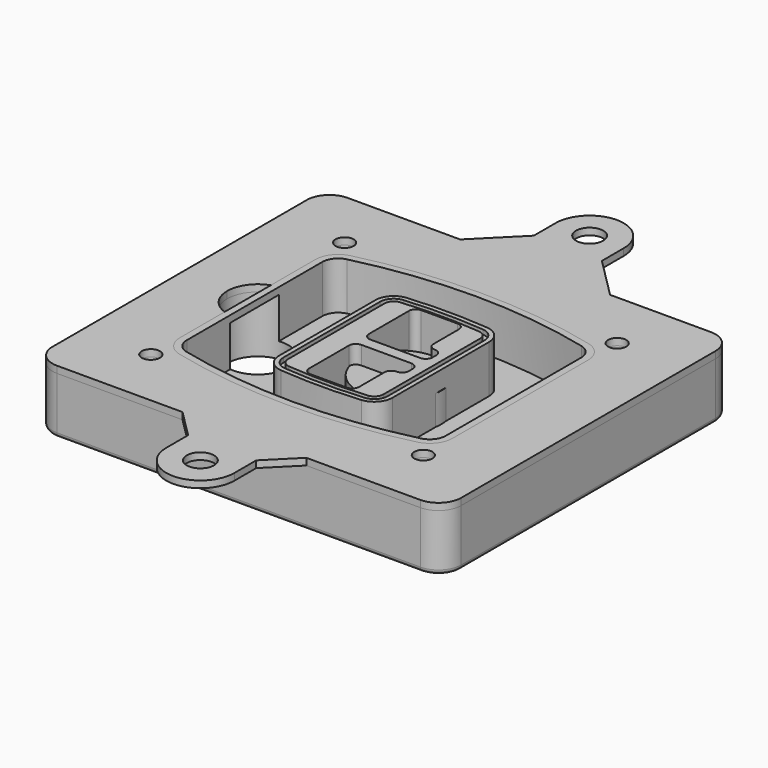
from build123d import *

# Parameters (mm, degrees)
F0_R      = 4
F1_DEPTH  = 25
F2_DEPTH  = 3
F3_DEPTH  = 18
F5_DEPTH  = 21
F6_DEPTH  = 2
F8_DEPTH  = 20
F9_DEPTH  = 16
F10_DEPTH = 25
F7_R      = 6
F7_R_2    = 4
F11_DEPTH = 6
F13_DEPTH = 9
F15_R     = 2
F16_R     = 6
F16_R_2   = 4
F17_DEPTH = 3


# Not quite as in the source:
# - a feature of the source that left no trace in its solid (it failed there, or was rolled back) is left out
# - a feature names something its author has since deleted; it is built from what else it names


with BuildPart() as f1:
    # F0 (on Top) → F1 (new body)
    with BuildSketch(Plane.XY):
        with BuildLine():
            ThreePointArc((-90, -70), (-87.0710678119, -77.0710678119), (-80, -80))
            Line((-80, -80), (80, -80))
            ThreePointArc((80, -80), (87.0710678119, -77.0710678119), (90, -70))
            Line((90, -70), (90, 70))
            ThreePointArc((90, 70), (87.0710678119, 77.0710678119), (80, 80))
            Line((80, 80), (-80, 80))
            ThreePointArc((-80, 80), (-87.0710678119, 77.0710678119), (-90, 70))
            Line((-90, 70), (-90, -70))
        make_face()
        with Locations((-60, -53.3333333333)):
            Circle(F0_R, mode=Mode.SUBTRACT)
        with Locations((60, -53.3333333333)):
            Circle(F0_R, mode=Mode.SUBTRACT)
        with Locations((-60, 53.3333333333)):
            Circle(F0_R, mode=Mode.SUBTRACT)
        with BuildLine():
            ThreePointArc((-64, 37.2990447398), (-61.0143011354, 45.9411029726), (-53.3306899286, 50.8970778549))
            ThreePointArc((-53.3306899286, 50.8970778549), (0, 57.3333333333), (53.3306899286, 50.8970778549))
            ThreePointArc((53.3306899286, 50.8970778549), (61.0143011354, 45.9411029726), (64, 37.2990447398))
            Line((64, 37.2990447398), (64, -37.2990447398))
            ThreePointArc((64, -37.2990447398), (61.0143011354, -45.9411029726), (53.3306899286, -50.8970778549))
            ThreePointArc((53.3306899286, -50.8970778549), (0, -57.3333333333), (-53.3306899286, -50.8970778549))
            ThreePointArc((-53.3306899286, -50.8970778549), (-61.0143011354, -45.9411029726), (-64, -37.2990447398))
            Line((-64, -37.2990447398), (-64, 37.2990447398))
        make_face(mode=Mode.SUBTRACT)
        with Locations((60, 53.3333333333)):
            Circle(F0_R, mode=Mode.SUBTRACT)
        with BuildLine():
            ThreePointArc((53.3306899286, 50.8970778549), (0, 57.3333333333), (-53.3306899286, 50.8970778549))
            ThreePointArc((-53.3306899286, 50.8970778549), (-61.0143011354, 45.9411029726), (-64, 37.2990447398))
            Line((-64, 37.2990447398), (-64, -37.2990447398))
            ThreePointArc((-64, -37.2990447398), (-61.0143011354, -45.9411029726), (-53.3306899286, -50.8970778549))
            ThreePointArc((-53.3306899286, -50.8970778549), (0, -57.3333333333), (53.3306899286, -50.8970778549))
            ThreePointArc((53.3306899286, -50.8970778549), (61.0143011354, -45.9411029726), (64, -37.2990447398))
            Line((64, -37.2990447398), (64, 37.2990447398))
            ThreePointArc((64, 37.2990447398), (61.0143011354, 45.9411029726), (53.3306899286, 50.8970778549))
        make_face()
        with BuildLine():
            Line((-60, -37.2990447398), (-60, 37.2990447398))
            ThreePointArc((-60, 37.2990447398), (-57.8673579538, 43.4719434775), (-52.3790642347, 47.0119255363))
            ThreePointArc((-52.3790642347, 47.0119255363), (0, 53.3333333333), (52.3790642347, 47.0119255363))
            ThreePointArc((52.3790642347, 47.0119255363), (57.8673579538, 43.4719434775), (60, 37.2990447398))
            Line((60, 37.2990447398), (60, -37.2990447398))
            ThreePointArc((60, -37.2990447398), (57.8673579538, -43.4719434775), (52.3790642347, -47.0119255363))
            ThreePointArc((52.3790642347, -47.0119255363), (0, -53.3333333333), (-52.3790642347, -47.0119255363))
            ThreePointArc((-52.3790642347, -47.0119255363), (-57.8673579538, -43.4719434775), (-60, -37.2990447398))
        make_face(mode=Mode.SUBTRACT)
        with BuildLine():
            ThreePointArc((-52.3790642347, 47.0119255363), (-57.8673579538, 43.4719434775), (-60, 37.2990447398))
            Line((-60, 37.2990447398), (-60, -37.2990447398))
            ThreePointArc((-60, -37.2990447398), (-57.8673579538, -43.4719434775), (-52.3790642347, -47.0119255363))
            ThreePointArc((-52.3790642347, -47.0119255363), (0, -53.3333333333), (52.3790642347, -47.0119255363))
            ThreePointArc((52.3790642347, -47.0119255363), (57.8673579538, -43.4719434775), (60, -37.2990447398))
            Line((60, -37.2990447398), (60, 37.2990447398))
            ThreePointArc((60, 37.2990447398), (57.8673579538, 43.4719434775), (52.3790642347, 47.0119255363))
            ThreePointArc((52.3790642347, 47.0119255363), (0, 53.3333333333), (-52.3790642347, 47.0119255363))
        make_face()
        with BuildLine():
            ThreePointArc((51.6653449643, 44.0980612973), (55.5071505677, 41.6200738562), (57, 37.2990447398))
            Line((57, 37.2990447398), (57, -37.2990447398))
            ThreePointArc((57, -37.2990447398), (55.5071505677, -41.6200738562), (51.6653449643, -44.0980612973))
            ThreePointArc((51.6653449643, -44.0980612973), (0, -50.3333333333), (-51.6653449643, -44.0980612973))
            ThreePointArc((-51.6653449643, -44.0980612973), (-55.5071505677, -41.6200738562), (-57, -37.2990447398))
            Line((-57, -37.2990447398), (-57, 37.2990447398))
            ThreePointArc((-57, 37.2990447398), (-55.5071505677, 41.6200738562), (-51.6653449643, 44.0980612973))
            ThreePointArc((-51.6653449643, 44.0980612973), (0, 50.3333333333), (51.6653449643, 44.0980612973))
        make_face(mode=Mode.SUBTRACT)
        with BuildLine():
            Line((57, -37.2990447398), (57, 37.2990447398))
            ThreePointArc((57, 37.2990447398), (55.5071505677, 41.6200738562), (51.6653449643, 44.0980612973))
            ThreePointArc((51.6653449643, 44.0980612973), (0, 50.3333333333), (-51.6653449643, 44.0980612973))
            ThreePointArc((-51.6653449643, 44.0980612973), (-55.5071505677, 41.6200738562), (-57, 37.2990447398))
            Line((-57, 37.2990447398), (-57, -37.2990447398))
            ThreePointArc((-57, -37.2990447398), (-55.5071505677, -41.6200738562), (-51.6653449643, -44.0980612973))
            ThreePointArc((-51.6653449643, -44.0980612973), (0, -50.3333333333), (51.6653449643, -44.0980612973))
            ThreePointArc((51.6653449643, -44.0980612973), (55.5071505677, -41.6200738562), (57, -37.2990447398))
        make_face()
    extrude(amount=-F1_DEPTH)

    # F0 (on Top) → F2 (join)
    with BuildSketch(Plane.XY):
        with BuildLine():
            ThreePointArc((-52.3790642347, 47.0119255363), (-57.8673579538, 43.4719434775), (-60, 37.2990447398))
            Line((-60, 37.2990447398), (-60, -37.2990447398))
            ThreePointArc((-60, -37.2990447398), (-57.8673579538, -43.4719434775), (-52.3790642347, -47.0119255363))
            ThreePointArc((-52.3790642347, -47.0119255363), (0, -53.3333333333), (52.3790642347, -47.0119255363))
            ThreePointArc((52.3790642347, -47.0119255363), (57.8673579538, -43.4719434775), (60, -37.2990447398))
            Line((60, -37.2990447398), (60, 37.2990447398))
            ThreePointArc((60, 37.2990447398), (57.8673579538, 43.4719434775), (52.3790642347, 47.0119255363))
            ThreePointArc((52.3790642347, 47.0119255363), (0, 53.3333333333), (-52.3790642347, 47.0119255363))
        make_face()
        with BuildLine():
            ThreePointArc((51.6653449643, 44.0980612973), (55.5071505677, 41.6200738562), (57, 37.2990447398))
            Line((57, 37.2990447398), (57, -37.2990447398))
            ThreePointArc((57, -37.2990447398), (55.5071505677, -41.6200738562), (51.6653449643, -44.0980612973))
            ThreePointArc((51.6653449643, -44.0980612973), (0, -50.3333333333), (-51.6653449643, -44.0980612973))
            ThreePointArc((-51.6653449643, -44.0980612973), (-55.5071505677, -41.6200738562), (-57, -37.2990447398))
            Line((-57, -37.2990447398), (-57, 37.2990447398))
            ThreePointArc((-57, 37.2990447398), (-55.5071505677, 41.6200738562), (-51.6653449643, 44.0980612973))
            ThreePointArc((-51.6653449643, 44.0980612973), (0, 50.3333333333), (51.6653449643, 44.0980612973))
        make_face(mode=Mode.SUBTRACT)
    extrude(amount=F2_DEPTH)

    # F0 (on Top) → F3 (cut)
    with BuildSketch(Plane.XY):
        with BuildLine():
            Line((57, -37.2990447398), (57, 37.2990447398))
            ThreePointArc((57, 37.2990447398), (55.5071505677, 41.6200738562), (51.6653449643, 44.0980612973))
            ThreePointArc((51.6653449643, 44.0980612973), (0, 50.3333333333), (-51.6653449643, 44.0980612973))
            ThreePointArc((-51.6653449643, 44.0980612973), (-55.5071505677, 41.6200738562), (-57, 37.2990447398))
            Line((-57, 37.2990447398), (-57, -37.2990447398))
            ThreePointArc((-57, -37.2990447398), (-55.5071505677, -41.6200738562), (-51.6653449643, -44.0980612973))
            ThreePointArc((-51.6653449643, -44.0980612973), (0, -50.3333333333), (51.6653449643, -44.0980612973))
            ThreePointArc((51.6653449643, -44.0980612973), (55.5071505677, -41.6200738562), (57, -37.2990447398))
        make_face()
    extrude(amount=-F3_DEPTH, mode=Mode.SUBTRACT)

    # F4 (on face) → F5 (join, through all)
    with BuildSketch(Plane.XY.offset(3)):
        with BuildLine():
            ThreePointArc((-25, -26.587695628), (-22.8992979869, -31.9912392117), (-17.7004291845, -34.5569740744))
            ThreePointArc((-17.7004291845, -34.5569740744), (0, -35.3333333333), (17.7004291845, -34.5569740744))
            ThreePointArc((17.7004291845, -34.5569740744), (22.8992979869, -31.9912392117), (25, -26.587695628))
            Line((25, -26.587695628), (25, 26.587695628))
            ThreePointArc((25, 26.587695628), (22.8992979869, 31.9912392117), (17.7004291845, 34.5569740744))
            ThreePointArc((17.7004291845, 34.5569740744), (0, 35.3333333333), (-17.7004291845, 34.5569740744))
            ThreePointArc((-17.7004291845, 34.5569740744), (-22.8992979869, 31.9912392117), (-25, 26.587695628))
            Line((-25, 26.587695628), (-25, -26.587695628))
        make_face()
        with BuildLine():
            ThreePointArc((17.5253218884, 32.5646544628), (21.4244734902, 30.6403533158), (23, 26.587695628))
            Line((23, 26.587695628), (23, -26.587695628))
            ThreePointArc((23, -26.587695628), (21.4244734902, -30.6403533158), (17.5253218884, -32.5646544628))
            ThreePointArc((17.5253218884, -32.5646544628), (0, -33.3333333333), (-17.5253218884, -32.5646544628))
            ThreePointArc((-17.5253218884, -32.5646544628), (-21.4244734902, -30.6403533158), (-23, -26.587695628))
            Line((-23, -26.587695628), (-23, 26.587695628))
            ThreePointArc((-23, 26.587695628), (-21.4244734902, 30.6403533158), (-17.5253218884, 32.5646544628))
            ThreePointArc((-17.5253218884, 32.5646544628), (0, 33.3333333333), (17.5253218884, 32.5646544628))
        make_face(mode=Mode.SUBTRACT)
        with BuildLine():
            Line((23, -26.587695628), (23, 26.587695628))
            ThreePointArc((23, 26.587695628), (21.4244734902, 30.6403533158), (17.5253218884, 32.5646544628))
            ThreePointArc((17.5253218884, 32.5646544628), (0, 33.3333333333), (-17.5253218884, 32.5646544628))
            ThreePointArc((-17.5253218884, 32.5646544628), (-21.4244734902, 30.6403533158), (-23, 26.587695628))
            Line((-23, 26.587695628), (-23, -26.587695628))
            ThreePointArc((-23, -26.587695628), (-21.4244734902, -30.6403533158), (-17.5253218884, -32.5646544628))
            ThreePointArc((-17.5253218884, -32.5646544628), (0, -33.3333333333), (17.5253218884, -32.5646544628))
            ThreePointArc((17.5253218884, -32.5646544628), (21.4244734902, -30.6403533158), (23, -26.587695628))
        make_face()
        with BuildLine():
            ThreePointArc((17.3502145923, 30.5723348512), (19.9496489934, 29.2894674198), (21, 26.587695628))
            Line((21, 26.587695628), (21, -26.587695628))
            ThreePointArc((21, -26.587695628), (19.9496489934, -29.2894674198), (17.3502145923, -30.5723348512))
            ThreePointArc((17.3502145923, -30.5723348512), (0, -31.3333333333), (-17.3502145923, -30.5723348512))
            ThreePointArc((-17.3502145923, -30.5723348512), (-19.9496489934, -29.2894674198), (-21, -26.587695628))
            Line((-21, -26.587695628), (-21, 26.587695628))
            ThreePointArc((-21, 26.587695628), (-19.9496489934, 29.2894674198), (-17.3502145923, 30.5723348512))
            ThreePointArc((-17.3502145923, 30.5723348512), (0, 31.3333333333), (17.3502145923, 30.5723348512))
        make_face(mode=Mode.SUBTRACT)
        with BuildLine():
            Line((21, -26.587695628), (21, 26.587695628))
            ThreePointArc((21, 26.587695628), (19.9496489934, 29.2894674198), (17.3502145923, 30.5723348512))
            ThreePointArc((17.3502145923, 30.5723348512), (0, 31.3333333333), (-17.3502145923, 30.5723348512))
            ThreePointArc((-17.3502145923, 30.5723348512), (-19.9496489934, 29.2894674198), (-21, 26.587695628))
            Line((-21, 26.587695628), (-21, -26.587695628))
            ThreePointArc((-21, -26.587695628), (-19.9496489934, -29.2894674198), (-17.3502145923, -30.5723348512))
            ThreePointArc((-17.3502145923, -30.5723348512), (0, -31.3333333333), (17.3502145923, -30.5723348512))
            ThreePointArc((17.3502145923, -30.5723348512), (19.9496489934, -29.2894674198), (21, -26.587695628))
        make_face()
        with BuildLine():
            Line((-8, -2.5), (14, -2.5))
            ThreePointArc((14, -2.5), (16.1213203436, -3.3786796564), (17, -5.5))
            Line((17, -5.5), (17, -7.5))
            ThreePointArc((17, -7.5), (16.1213203436, -9.6213203436), (14, -10.5))
            ThreePointArc((14, -10.5), (11.8786796564, -11.3786796564), (11, -13.5))
            Line((11, -13.5), (11, -27.5))
            ThreePointArc((11, -27.5), (10.1213203436, -29.6213203436), (8, -30.5))
            Line((8, -30.5), (-8, -30.5))
            ThreePointArc((-8, -30.5), (-10.1213203436, -29.6213203436), (-11, -27.5))
            Line((-11, -27.5), (-11, -5.5))
            ThreePointArc((-11, -5.5), (-10.1213203436, -3.3786796564), (-8, -2.5))
        make_face(mode=Mode.SUBTRACT)
        with BuildLine():
            ThreePointArc((-8, 2.5), (-10.1213203436, 3.3786796564), (-11, 5.5))
            Line((-11, 5.5), (-11, 27.5))
            ThreePointArc((-11, 27.5), (-10.1213203436, 29.6213203436), (-8, 30.5))
            Line((-8, 30.5), (8, 30.5))
            ThreePointArc((8, 30.5), (10.1213203436, 29.6213203436), (11, 27.5))
            Line((11, 27.5), (11, 13.5))
            ThreePointArc((11, 13.5), (11.8786796564, 11.3786796564), (14, 10.5))
            ThreePointArc((14, 10.5), (16.1213203436, 9.6213203436), (17, 7.5))
            Line((17, 7.5), (17, 5.5))
            ThreePointArc((17, 5.5), (16.1213203436, 3.3786796564), (14, 2.5))
            Line((14, 2.5), (-8, 2.5))
        make_face(mode=Mode.SUBTRACT)
    extrude(amount=-F5_DEPTH)

    # F4 (on face) → F6 (cut)
    with BuildSketch(Plane.XY.offset(3)):
        with BuildLine():
            Line((23, -26.587695628), (23, 26.587695628))
            ThreePointArc((23, 26.587695628), (21.4244734902, 30.6403533158), (17.5253218884, 32.5646544628))
            ThreePointArc((17.5253218884, 32.5646544628), (0, 33.3333333333), (-17.5253218884, 32.5646544628))
            ThreePointArc((-17.5253218884, 32.5646544628), (-21.4244734902, 30.6403533158), (-23, 26.587695628))
            Line((-23, 26.587695628), (-23, -26.587695628))
            ThreePointArc((-23, -26.587695628), (-21.4244734902, -30.6403533158), (-17.5253218884, -32.5646544628))
            ThreePointArc((-17.5253218884, -32.5646544628), (0, -33.3333333333), (17.5253218884, -32.5646544628))
            ThreePointArc((17.5253218884, -32.5646544628), (21.4244734902, -30.6403533158), (23, -26.587695628))
        make_face()
        with BuildLine():
            ThreePointArc((17.3502145923, 30.5723348512), (19.9496489934, 29.2894674198), (21, 26.587695628))
            Line((21, 26.587695628), (21, -26.587695628))
            ThreePointArc((21, -26.587695628), (19.9496489934, -29.2894674198), (17.3502145923, -30.5723348512))
            ThreePointArc((17.3502145923, -30.5723348512), (0, -31.3333333333), (-17.3502145923, -30.5723348512))
            ThreePointArc((-17.3502145923, -30.5723348512), (-19.9496489934, -29.2894674198), (-21, -26.587695628))
            Line((-21, -26.587695628), (-21, 26.587695628))
            ThreePointArc((-21, 26.587695628), (-19.9496489934, 29.2894674198), (-17.3502145923, 30.5723348512))
            ThreePointArc((-17.3502145923, 30.5723348512), (0, 31.3333333333), (17.3502145923, 30.5723348512))
        make_face(mode=Mode.SUBTRACT)
    extrude(amount=-F6_DEPTH, mode=Mode.SUBTRACT)

    # F7 (on face) → F8 (join)
    with BuildSketch(Plane(origin=(0, 0, -25), x_dir=(1, 0, 0), z_dir=(0, 0, -1))):
        with BuildLine():
            ThreePointArc((-6.71157564, 0), (6.7567035675, 13.4682792075), (20.224982775, 0))
            Line((20.224982775, 0), (25.224982775, 0))
            ThreePointArc((25.224982775, 0), (6.7567035675, 18.4682792075), (-11.71157564, 0))
            Line((-11.71157564, 0), (-6.71157564, 0))
        make_face()
        with BuildLine():
            Line((-6.71157564, 0), (20.224982775, 0))
            ThreePointArc((20.224982775, 0), (6.7567035675, 13.4682792075), (-6.71157564, 0))
        make_face()
        with BuildLine():
            ThreePointArc((-6.71157564, 0), (6.7567035675, -13.4682792075), (20.224982775, 0))
            Line((20.224982775, 0), (-6.71157564, 0))
        make_face()
        with BuildLine():
            Line((25.224982775, 0), (20.224982775, 0))
            ThreePointArc((20.224982775, 0), (6.7567035675, -13.4682792075), (-6.71157564, 0))
            Line((-6.71157564, 0), (-11.71157564, 0))
            ThreePointArc((-11.71157564, 0), (6.7567035675, -18.4682792075), (25.224982775, 0))
        make_face()
    extrude(amount=-F8_DEPTH)

    # F7 (on face) → F9 (cut)
    with BuildSketch(Plane(origin=(0, 0, -25), x_dir=(1, 0, 0), z_dir=(0, 0, -1))):
        with BuildLine():
            Line((-6.71157564, 0), (20.224982775, 0))
            ThreePointArc((20.224982775, 0), (6.7567035675, 13.4682792075), (-6.71157564, 0))
        make_face()
        with BuildLine():
            ThreePointArc((-6.71157564, 0), (6.7567035675, -13.4682792075), (20.224982775, 0))
            Line((20.224982775, 0), (-6.71157564, 0))
        make_face()
    extrude(amount=-F9_DEPTH, mode=Mode.SUBTRACT)

    # F7 (on face) → F10 (cut)
    with BuildSketch(Plane(origin=(0, 0, -25), x_dir=(1, 0, 0), z_dir=(0, 0, -1))):
        with BuildLine():
            Line((-69.0318229325, 0), (-42.0952645175, 0))
            ThreePointArc((-42.0952645175, 0), (-55.563543725, 13.4682792075), (-69.0318229325, 0))
        make_face()
        with BuildLine():
            ThreePointArc((-69.0318229325, 0), (-55.563543725, -13.4682792075), (-42.0952645175, 0))
            Line((-42.0952645175, 0), (-69.0318229325, 0))
        make_face()
    extrude(amount=-F10_DEPTH, mode=Mode.SUBTRACT)

    # F7 (on face) → F11 (cut)
    with BuildSketch(Plane(origin=(0, 0, -25), x_dir=(1, 0, 0), z_dir=(0, 0, -1))):
        with Locations((60, -53.3333333333)):
            Circle(F7_R)
        with Locations((60, -53.3333333333)):
            Circle(F7_R_2, mode=Mode.SUBTRACT)
        with Locations((-60, -53.3333333333)):
            Circle(F7_R)
        with Locations((-60, -53.3333333333)):
            Circle(F7_R_2, mode=Mode.SUBTRACT)
        with Locations((-60, 53.3333333333)):
            Circle(F7_R)
        with Locations((-60, 53.3333333333)):
            Circle(F7_R_2, mode=Mode.SUBTRACT)
        with Locations((60, 53.3333333333)):
            Circle(F7_R)
        with Locations((60, 53.3333333333)):
            Circle(F7_R_2, mode=Mode.SUBTRACT)
    extrude(amount=-F11_DEPTH, mode=Mode.SUBTRACT)

    # F12 (on face) → F13 (cut, through all)
    with BuildSketch(Plane(origin=(0, 0, -9), x_dir=(1, 0, 0), z_dir=(0, 0, -1))):
        with BuildLine():
            ThreePointArc((20.224982775, 0), (20.1663399806, 1.2554664788), (19.9909222755, 2.5))
            Line((19.9909222755, 2.5), (14, 2.5))
            ThreePointArc((14, 2.5), (16.1213203436, 3.3786796564), (17, 5.5))
            Line((17, 5.5), (17, 7.5))
            ThreePointArc((17, 7.5), (16.1213203436, 9.6213203436), (14, 10.5))
            ThreePointArc((14, 10.5), (12.1627255951, 11.1284134507), (11.0951631559, 12.750384826))
            ThreePointArc((11.0951631559, 12.750384826), (11.0476113807, 12.7664660322), (11, 12.7823698976))
            Line((11, 12.7823698976), (11, -12.7823698976))
            ThreePointArc((11, -12.7823698976), (11.0476113807, -12.7664660322), (11.0951631559, -12.750384826))
            ThreePointArc((11.0951631559, -12.750384826), (12.1627255951, -11.1284134507), (14, -10.5))
            ThreePointArc((14, -10.5), (16.1213203436, -9.6213203436), (17, -7.5))
            Line((17, -7.5), (17, -5.5))
            ThreePointArc((17, -5.5), (16.1213203436, -3.3786796564), (14, -2.5))
            Line((14, -2.5), (19.9909222755, -2.5))
            ThreePointArc((19.9909222755, -2.5), (20.1663399806, -1.2554664788), (20.224982775, 0))
        make_face()
    extrude(amount=F13_DEPTH, mode=Mode.SUBTRACT)

    # F15
    f15_edges = [f1.edges().sort_by_distance(p)[0] for p in [
        (0, -80, -25),
        (-87.071068, -77.071068, -25),
        (-90, 0, -25),
        (-87.071068, 77.071068, -25),
        (87.071068, -77.071068, -25),
        (0, 80, -25),
        (90, 0, -25),
        (87.071068, 77.071068, -25),
    ]]
    fillet(f15_edges, radius=F15_R)


with BuildPart() as f17:
    # F16 (on face) → F17 (new body, through all)
    with BuildSketch(Plane.XY):
        with BuildLine():
            Line((-12.457734853, 98), (-30.457734853, 80))
            Line((-30.457734853, 80), (35.542265147, 80))
            Line((35.542265147, 80), (17.542265147, 98))
            Line((17.542265147, 98), (17.542265147, 110))
            ThreePointArc((17.542265147, 110), (2.542265147, 125), (-12.457734853, 110))
            Line((-12.457734853, 110), (-12.457734853, 98))
        make_face()
        with Locations((2.542265147, 110)):
            Circle(F16_R, mode=Mode.SUBTRACT)
        with BuildLine():
            Line((35.542265147, 80), (-30.457734853, 80))
            Line((-30.457734853, 80), (-80, 80))
            ThreePointArc((-80, 80), (-87.0710678119, 77.0710678119), (-90, 70))
            Line((-90, 70), (-90, -70))
            ThreePointArc((-90, -70), (-87.0710678119, -77.0710678119), (-80, -80))
            Line((-80, -80), (-24.707734853, -80))
            Line((-24.707734853, -80), (29.792265147, -80))
            Line((29.792265147, -80), (80, -80))
            ThreePointArc((80, -80), (87.0710678119, -77.0710678119), (90, -70))
            Line((90, -70), (90, 70))
            ThreePointArc((90, 70), (87.0710678119, 77.0710678119), (80, 80))
            Line((80, 80), (35.542265147, 80))
        make_face()
        with Locations((-60, -53.3333333333)):
            Circle(F16_R_2, mode=Mode.SUBTRACT)
        with BuildLine():
            Line((-60, 12.7166190685), (-60, 37.2990447398))
            ThreePointArc((-60, 37.2990447398), (-57.8673579538, 43.4719434775), (-52.3790642347, 47.0119255363))
            ThreePointArc((-52.3790642347, 47.0119255363), (0, 53.3333333333), (52.3790642347, 47.0119255363))
            ThreePointArc((52.3790642347, 47.0119255363), (57.8673579538, 43.4719434775), (60, 37.2990447398))
            Line((60, 37.2990447398), (60, -37.2990447398))
            ThreePointArc((60, -37.2990447398), (57.8673579538, -43.4719434775), (52.3790642347, -47.0119255363))
            ThreePointArc((52.3790642347, -47.0119255363), (0, -53.3333333333), (-52.3790642347, -47.0119255363))
            ThreePointArc((-52.3790642347, -47.0119255363), (-57.8673579538, -43.4719434775), (-60, -37.2990447398))
            Line((-60, -37.2990447398), (-60, -12.7166190685))
            ThreePointArc((-60, -12.7166190685), (-66.5441169481, -7.798817635), (-69.0318229325, 0))
            ThreePointArc((-69.0318229325, 0), (-66.5441169481, 7.798817635), (-60, 12.7166190685))
        make_face(mode=Mode.SUBTRACT)
        with Locations((60, -53.3333333333)):
            Circle(F16_R_2, mode=Mode.SUBTRACT)
        with Locations((-60, 53.3333333333)):
            Circle(F16_R_2, mode=Mode.SUBTRACT)
        with Locations((60, 53.3333333333)):
            Circle(F16_R_2, mode=Mode.SUBTRACT)
        with BuildLine():
            Line((29.792265147, -80), (-24.707734853, -80))
            Line((-24.707734853, -80), (-12.457734853, -92.25))
            Line((-12.457734853, -92.25), (-12.457734853, -104.25))
            ThreePointArc((-12.457734853, -104.25), (2.542265147, -119.25), (17.542265147, -104.25))
            Line((17.542265147, -104.25), (17.542265147, -92.25))
            Line((17.542265147, -92.25), (29.792265147, -80))
        make_face()
        with Locations((2.542265147, -104.25)):
            Circle(F16_R, mode=Mode.SUBTRACT)
    extrude(amount=F17_DEPTH)


solid = Compound([f1.part, f17.part])
